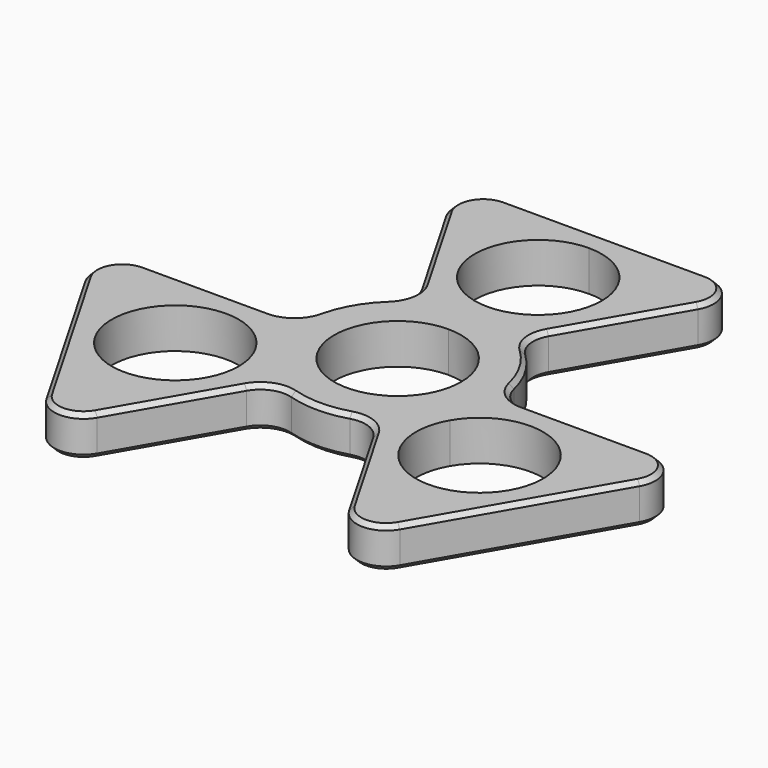
from build123d import *

# Parameters (mm, degrees)
F1_DEPTH = 6.985
F2_R     = 5.08
F3_SIZE  = 0.762


with BuildPart() as f1:
    # F0 (on Top) → F1 (new body)
    with BuildSketch(Plane.XY):
        with BuildLine():
            ThreePointArc((-7.41045, 12.8352759069), (-3.8359311856, 14.3158900788), (0, 14.8209))
            Line((0, 14.8209), (0, 17.4625))
            ThreePointArc((0, 17.4625), (-4.5196275751, 16.8674797416), (-8.73125, 15.1229686136))
            Line((-8.73125, 15.1229686136), (-7.41045, 12.8352759069))
        make_face()
        with BuildLine():
            Line((0, 17.4625), (0, 14.8209))
            ThreePointArc((0, 14.8209), (3.8359311856, 14.3158900788), (7.41045, 12.8352759069))
            Line((7.41045, 12.8352759069), (8.73125, 15.1229686136))
            ThreePointArc((8.73125, 15.1229686136), (4.5196275751, 16.8674797416), (0, 17.4625))
        make_face()
        with BuildLine():
            ThreePointArc((14.8209, 0), (14.3158900788, -3.8359311856), (12.8352759069, -7.41045))
            Line((12.8352759069, -7.41045), (15.1229686136, -8.73125))
            ThreePointArc((15.1229686136, -8.73125), (16.8674797416, -4.5196275751), (17.4625, 0))
            Line((17.4625, 0), (14.8209, 0))
        make_face()
        with BuildLine():
            Line((15.1229686136, -8.73125), (12.8352759069, -7.41045))
            ThreePointArc((12.8352759069, -7.41045), (10.4799588933, -10.4799588933), (7.41045, -12.8352759069))
            Line((7.41045, -12.8352759069), (8.73125, -15.1229686136))
            ThreePointArc((8.73125, -15.1229686136), (12.3478521665, -12.3478521665), (15.1229686136, -8.73125))
        make_face()
        with BuildLine():
            ThreePointArc((-7.41045, -12.8352759069), (-10.4799588933, -10.4799588933), (-12.8352759069, -7.41045))
            Line((-12.8352759069, -7.41045), (-15.1229686136, -8.73125))
            ThreePointArc((-15.1229686136, -8.73125), (-12.3478521665, -12.3478521665), (-8.73125, -15.1229686136))
            Line((-8.73125, -15.1229686136), (-7.41045, -12.8352759069))
        make_face()
        with BuildLine():
            Line((-15.1229686136, -8.73125), (-12.8352759069, -7.41045))
            ThreePointArc((-12.8352759069, -7.41045), (-14.3158900788, -3.8359311856), (-14.8209, 0))
            Line((-14.8209, 0), (-17.4625, 0))
            ThreePointArc((-17.4625, 0), (-16.8674797416, -4.5196275751), (-15.1229686136, -8.73125))
        make_face()
        with BuildLine():
            ThreePointArc((-8.73125, 15.1229686136), (-4.5196275751, 16.8674797416), (0, 17.4625))
            Line((0, 17.4625), (0, 19.4691))
            ThreePointArc((0, 19.4691), (-11.0109, 30.48), (0, 41.4909))
            Line((0, 41.4909), (0, 45.466))
            Line((0, 45.466), (-26.249807339, 45.466))
            Line((-26.249807339, 45.466), (-8.73125, 15.1229686136))
        make_face()
        with BuildLine():
            Line((0, 19.4691), (0, 17.4625))
            ThreePointArc((0, 17.4625), (4.5196275751, 16.8674797416), (8.73125, 15.1229686136))
            Line((8.73125, 15.1229686136), (26.249807339, 45.466))
            Line((26.249807339, 45.466), (0, 45.466))
            Line((0, 45.466), (0, 41.4909))
            ThreePointArc((0, 41.4909), (7.785882057, 38.265882057), (11.0109, 30.48))
            ThreePointArc((11.0109, 30.48), (7.785882057, 22.694117943), (0, 19.4691))
        make_face()
        with BuildLine():
            Line((8.73125, 15.1229686136), (7.41045, 12.8352759069))
            ThreePointArc((7.41045, 12.8352759069), (12.8352759069, 7.41045), (14.8209, 0))
            Line((14.8209, 0), (17.4625, 0))
            ThreePointArc((17.4625, 0), (15.1229686136, 8.73125), (8.73125, 15.1229686136))
        make_face()
        with BuildLine():
            ThreePointArc((-14.8209, 0), (-12.8352759069, 7.41045), (-7.41045, 12.8352759069))
            Line((-7.41045, 12.8352759069), (-8.73125, 15.1229686136))
            ThreePointArc((-8.73125, 15.1229686136), (-15.1229686136, 8.73125), (-17.4625, 0))
            Line((-17.4625, 0), (-14.8209, 0))
        make_face()
        with BuildLine():
            ThreePointArc((17.4625, 0), (16.8674797416, -4.5196275751), (15.1229686136, -8.73125))
            Line((15.1229686136, -8.73125), (16.8607351888, -9.73455))
            ThreePointArc((16.8607351888, -9.73455), (29.2462849311, -4.6042873193), (37.4073543073, -15.24))
            ThreePointArc((37.4073543073, -15.24), (37.032166988, -18.0898306237), (35.9321734259, -20.74545))
            Line((35.9321734259, -20.74545), (39.3747110085, -22.733))
            Line((39.3747110085, -22.733), (52.499614678, 0))
            Line((52.499614678, 0), (17.4625, 0))
        make_face()
        with BuildLine():
            Line((16.8607351888, -9.73455), (15.1229686136, -8.73125))
            ThreePointArc((15.1229686136, -8.73125), (12.3478521665, -12.3478521665), (8.73125, -15.1229686136))
            Line((8.73125, -15.1229686136), (26.249807339, -45.466))
            Line((26.249807339, -45.466), (39.3747110085, -22.733))
            Line((39.3747110085, -22.733), (35.9321734259, -20.74545))
            ThreePointArc((35.9321734259, -20.74545), (20.8910043073, -24.7757191185), (16.8607351888, -9.73455))
        make_face()
        with BuildLine():
            Line((8.73125, -15.1229686136), (7.41045, -12.8352759069))
            ThreePointArc((7.41045, -12.8352759069), (0, -14.8209), (-7.41045, -12.8352759069))
            Line((-7.41045, -12.8352759069), (-8.73125, -15.1229686136))
            ThreePointArc((-8.73125, -15.1229686136), (0, -17.4625), (8.73125, -15.1229686136))
        make_face()
        with BuildLine():
            ThreePointArc((-8.73125, -15.1229686136), (-12.3478521665, -12.3478521665), (-15.1229686136, -8.73125))
            Line((-15.1229686136, -8.73125), (-16.8607351888, -9.73455))
            ThreePointArc((-16.8607351888, -9.73455), (-15.7607416267, -12.3901693763), (-15.3855543073, -15.24))
            ThreePointArc((-15.3855543073, -15.24), (-23.5466236836, -25.8757126807), (-35.9321734259, -20.74545))
            Line((-35.9321734259, -20.74545), (-39.3747110085, -22.733))
            Line((-39.3747110085, -22.733), (-26.249807339, -45.466))
            Line((-26.249807339, -45.466), (-8.73125, -15.1229686136))
        make_face()
        with BuildLine():
            Line((-16.8607351888, -9.73455), (-15.1229686136, -8.73125))
            ThreePointArc((-15.1229686136, -8.73125), (-16.8674797416, -4.5196275751), (-17.4625, 0))
            Line((-17.4625, 0), (-52.499614678, 0))
            Line((-52.499614678, 0), (-39.3747110085, -22.733))
            Line((-39.3747110085, -22.733), (-35.9321734259, -20.74545))
            ThreePointArc((-35.9321734259, -20.74545), (-31.9019043073, -5.7042808815), (-16.8607351888, -9.73455))
        make_face()
        with BuildLine():
            ThreePointArc((-9.5357191185, -5.50545), (-9.5357191185, 5.50545), (0, 11.0109))
            Line((0, 11.0109), (0, 14.8209))
            ThreePointArc((0, 14.8209), (-3.8359311856, 14.3158900788), (-7.41045, 12.8352759069))
            ThreePointArc((-7.41045, 12.8352759069), (-12.8352759069, 7.41045), (-14.8209, 0))
            ThreePointArc((-14.8209, 0), (-14.3158900788, -3.8359311856), (-12.8352759069, -7.41045))
            Line((-12.8352759069, -7.41045), (-9.5357191185, -5.50545))
        make_face()
        with BuildLine():
            ThreePointArc((0, 11.0109), (7.785882057, 7.785882057), (11.0109, 0))
            ThreePointArc((11.0109, 0), (10.6357126807, -2.8498306237), (9.5357191185, -5.50545))
            Line((9.5357191185, -5.50545), (12.8352759069, -7.41045))
            ThreePointArc((12.8352759069, -7.41045), (14.3158900788, -3.8359311856), (14.8209, 0))
            ThreePointArc((14.8209, 0), (12.8352759069, 7.41045), (7.41045, 12.8352759069))
            ThreePointArc((7.41045, 12.8352759069), (3.8359311856, 14.3158900788), (0, 14.8209))
            Line((0, 14.8209), (0, 11.0109))
        make_face()
        with BuildLine():
            Line((12.8352759069, -7.41045), (9.5357191185, -5.50545))
            ThreePointArc((9.5357191185, -5.50545), (0, -11.0109), (-9.5357191185, -5.50545))
            Line((-9.5357191185, -5.50545), (-12.8352759069, -7.41045))
            ThreePointArc((-12.8352759069, -7.41045), (-10.4799588933, -10.4799588933), (-7.41045, -12.8352759069))
            ThreePointArc((-7.41045, -12.8352759069), (0, -14.8209), (7.41045, -12.8352759069))
            ThreePointArc((7.41045, -12.8352759069), (10.4799588933, -10.4799588933), (12.8352759069, -7.41045))
        make_face()
    extrude(amount=F1_DEPTH)

    # F2
    f2_edges = [f1.edges().sort_by_distance(p)[0] for p in [
        (8.73125, -15.122969, 3.4925),
        (26.249807, -45.466, 3.4925),
        (52.499615, 0, 3.4925),
        (17.4625, 0, 3.4925),
        (8.73125, 15.122969, 3.4925),
        (26.249807, 45.466, 3.4925),
        (-26.249807, 45.466, 3.4925),
        (-8.73125, 15.122969, 3.4925),
        (-17.4625, 0, 3.4925),
        (-52.499615, 0, 3.4925),
        (-26.249807, -45.466, 3.4925),
        (-8.73125, -15.122969, 3.4925),
    ]]
    fillet(f2_edges, radius=F2_R)

    # F3
    f3_edges = [f1.edges().sort_by_distance(p)[0] for p in [
        (-32.831722, 0, 6.985),
        (-16.415861, 28.433106, 6.985),
        (32.831722, 0, 6.985),
        (16.415861, 28.433106, 6.985),
        (0, 45.466, 6.985),
        (-39.374711, -22.733, 6.985),
        (39.374711, -22.733, 6.985),
        (16.415861, -28.433106, 6.985),
        (-16.415861, -28.433106, 6.985),
        (-16.415861, -28.433106, 0),
        (-32.831722, 0, 0),
        (-16.415861, 28.433106, 0),
        (16.415861, 28.433106, 0),
        (32.831722, 0, 0),
        (16.415861, -28.433106, 0),
        (39.374711, -22.733, 0),
        (0, 45.466, 0),
        (-39.374711, -22.733, 0),
        (8.444714, -16.834073, 0),
        (26.249807, -40.386, 0),
        (0, -17.4625, 0),
        (-8.444714, -16.834073, 0),
        (48.100206, -2.54, 0),
        (-26.249807, -40.386, 0),
        (18.801092, 1.1037, 0),
        (15.122969, 8.73125, 0),
        (-48.100206, -2.54, 0),
        (10.356378, 15.730373, 0),
        (-18.801092, 1.1037, 0),
        (21.850398, 42.926, 0),
        (-15.122969, 8.73125, 0),
        (-10.356378, 15.730373, 0),
        (-21.850398, 42.926, 0),
        (8.444714, -16.834073, 6.985),
        (26.249807, -40.386, 6.985),
        (0, -17.4625, 6.985),
        (-8.444714, -16.834073, 6.985),
        (48.100206, -2.54, 6.985),
        (-26.249807, -40.386, 6.985),
        (18.801092, 1.1037, 6.985),
        (15.122969, 8.73125, 6.985),
        (-48.100206, -2.54, 6.985),
        (10.356378, 15.730373, 6.985),
        (-18.801092, 1.1037, 6.985),
        (21.850398, 42.926, 6.985),
        (-15.122969, 8.73125, 6.985),
        (-10.356378, 15.730373, 6.985),
        (-21.850398, 42.926, 6.985),
    ]]
    chamfer(f3_edges, length=F3_SIZE)


solid = f1.part
